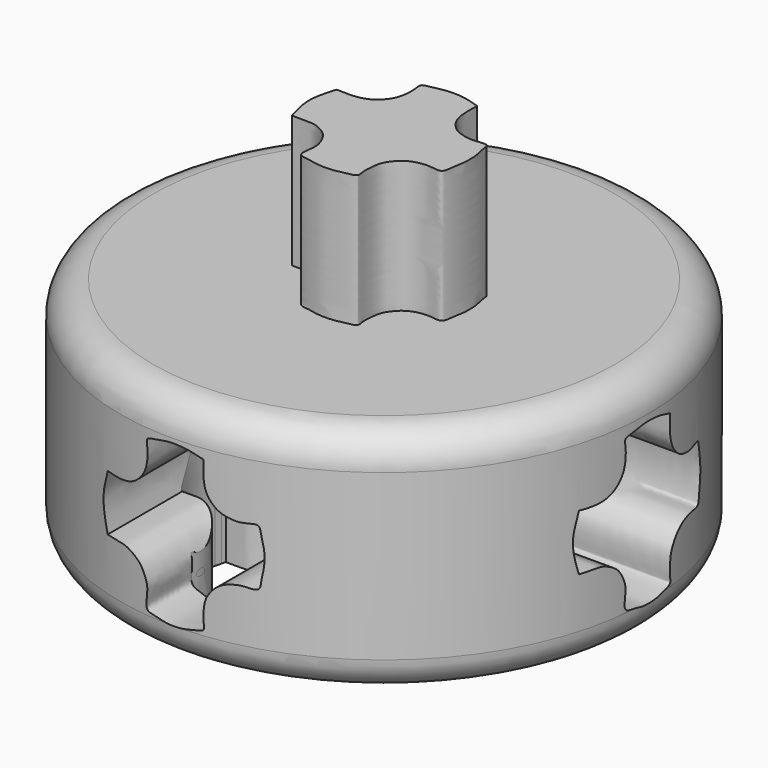
from build123d import *

# Parameters (mm, degrees)
F0_R          = 8
F1_DEPTH      = 7
F3_DEPTH      = 4
F5_DEPTH      = 25
F5_DEPTH_BACK = 25
F7_DEPTH      = 25
F7_DEPTH_BACK = 25
F9_DEPTH      = 5


# Not quite as in the source:
# - a fillet or chamfer that OpenCascade refuses, or shapes differently, is made with other operations: its cross-section is extruded or revolved along the edge and cut away or added


with BuildPart() as f1:
    # F0 (on Top) → F1 (new body)
    with BuildSketch(Plane.XY):
        Circle(F0_R)
    extrude(amount=F1_DEPTH)

    # F2 (on face) → F3 (join)
    with BuildSketch(Plane.XY.offset(7)):
        with BuildLine():
            add(Edge.make_bspline(
                [(-2.1453189292, -0.812403534), (-2.2291799027, -0.5147854162), (-2.3965988205, 0.0693154166), (-2.2270661408, 0.6183251281), (-2.1453189292, 0.8875972993)],
                knots=[0, 0, 0, 0, 0.5095712537, 1, 1, 1, 1], degree=3))
            add(Edge.make_bspline(
                [(-2.1453189292, -0.812403534), (-2.0462146869, -0.812546633), (-1.8562976232, -0.8128208589), (-1.5995258635, -0.8109702484), (-1.4107650431, -0.8271952097), (-1.0525308973, -0.9991228135), (-0.881515203, -1.2019496068), (-0.7462403154, -1.4790785152), (-0.6941521408, -1.7721486922), (-0.8264550317, -2.3060372512), (-0.4252380891, -2.3094553952), (-0.1641394597, -2.39328354), (0.171847139, -2.4065584213), (0.4619958492, -2.3819187352), (0.7053356837, -2.3086277115), (1.0355815173, -2.2738283861), (0.9578656682, -2.0264843097), (0.972329852, -1.7262282264), (1.0043166569, -1.4743095735), (1.0802938039, -1.2844806936), (1.2606264856, -1.0560642251), (1.4022161443, -0.9536037149), (1.5820445887, -0.8553488053), (1.8405387734, -0.8091796541), (2.0652910938, -0.7963302445), (2.4574534093, -0.8884051228), (2.4647792182, -0.5364288415), (2.5502262108, -0.2130675085), (2.5516869242, 0.0734966508), (2.5466202723, 0.3368604343), (2.4464405951, 0.6869113476), (2.4458836528, 0.9477445076), (2.0587086229, 0.8750622393), (1.8110087922, 0.8774528734), (1.460553932, 0.9794284484), (1.2720689076, 1.1213458505), (1.039296652, 1.3914645052), (0.9576696828, 1.8177575628), (0.969636174, 2.1409695187), (0.9758471819, 2.3087272993)],
                knots=[0, 0, 0, 0, 0.0273605905, 0.0524320947, 0.0745076412, 0.1056108167, 0.1318649214, 0.158948127, 0.1874687016, 0.220995097, 0.2482860623, 0.2755720453, 0.3045111481, 0.3315301836, 0.3578655515, 0.3837385363, 0.4059679792, 0.434252013, 0.4594532962, 0.4822711791, 0.5090972104, 0.530231005, 0.5527300135, 0.5781274322, 0.6031996615, 0.6315546276, 0.6576667534, 0.6876672756, 0.714256594, 0.7402463844, 0.7710533559, 0.7932728015, 0.8216277676, 0.8482190477, 0.8777914221, 0.9023565188, 0.9315770045, 0.9644861842, 1, 1, 1, 1], degree=3))
            add(Edge.make_bspline(
                [(-2.1453189292, 0.8875972993), (-1.9521964497, 0.8780475085), (-1.5848074134, 0.8603693676), (-1.1304602567, 0.9960226139), (-0.8202192306, 1.3400161654), (-0.7149185223, 1.6828007485), (-0.70557119, 2.0923268409), (-0.7793227574, 2.3463238004), (-0.4576002352, 2.3842425435), (-0.1008664347, 2.4800264396), (0.2451665152, 2.4783343449), (0.5684540927, 2.4417658867), (0.8334725478, 2.3546593956), (0.9758471819, 2.3087272993)],
                knots=[0, 0, 0, 0, 0.1117445823, 0.2125923647, 0.3107430927, 0.4000660841, 0.4960442665, 0.5626441507, 0.6379036869, 0.7311412958, 0.8178947498, 0.9022950941, 1, 1, 1, 1], degree=3))
        make_face()
    extrude(amount=F3_DEPTH)

    # F4 (on Right) → F5 (cut, two sides)
    with BuildSketch(Plane.YZ) as f5_sk:
        with BuildLine():
            add(Edge.make_bspline(
                [(-2.2211652576, 2.5211653882), (-2.3050262311, 2.8187835061), (-2.4724451489, 3.4028843389), (-2.3029124692, 3.9518940503), (-2.2211652576, 4.2211662216)],
                knots=[0, 0, 0, 0, 0.5095712537, 1, 1, 1, 1], degree=3))
            add(Edge.make_bspline(
                [(-2.2211652576, 2.5211653882), (-2.1220610153, 2.5210222892), (-1.9321439516, 2.5207480634), (-1.6753721919, 2.5225986738), (-1.4866113715, 2.5063737125), (-1.1283772257, 2.3344461087), (-0.9573615314, 2.1316193155), (-0.8220866438, 1.854490407), (-0.7699984692, 1.56142023), (-0.9023013601, 1.0275316711), (-0.5010844175, 1.024113527), (-0.2399857881, 0.9402853822), (0.0960008106, 0.927010501), (0.3861495208, 0.951650187), (0.6294893553, 1.0249412107), (0.9597351889, 1.0597405361), (0.8820193398, 1.3070846125), (0.8964835236, 1.6073406958), (0.9284703285, 1.8592593487), (1.0044474755, 2.0490882286), (1.1847801572, 2.2775046971), (1.3263698159, 2.3799652073), (1.5061982603, 2.478220117), (1.764692445, 2.5243892682), (1.9894447654, 2.5372386778), (2.3816070809, 2.4451637994), (2.3889328898, 2.7971400808), (2.4743798824, 3.1205014137), (2.4758405958, 3.4070655731), (2.4707739439, 3.6704293566), (2.3705942667, 4.0204802698), (2.3700373244, 4.2813134299), (1.9828622945, 4.2086311615), (1.7351624638, 4.2110217957), (1.3847076036, 4.3129973707), (1.1962225792, 4.4549147728), (0.9634503236, 4.7250334274), (0.8818233544, 5.1513264851), (0.8937898456, 5.4745384409), (0.9000008535, 5.6422962216)],
                knots=[0, 0, 0, 0, 0.0273605905, 0.0524320947, 0.0745076412, 0.1056108167, 0.1318649214, 0.158948127, 0.1874687016, 0.220995097, 0.2482860623, 0.2755720453, 0.3045111481, 0.3315301836, 0.3578655515, 0.3837385363, 0.4059679792, 0.434252013, 0.4594532962, 0.4822711791, 0.5090972104, 0.530231005, 0.5527300135, 0.5781274322, 0.6031996615, 0.6315546276, 0.6576667534, 0.6876672756, 0.714256594, 0.7402463844, 0.7710533559, 0.7932728015, 0.8216277676, 0.8482190477, 0.8777914221, 0.9023565188, 0.9315770045, 0.9644861842, 1, 1, 1, 1], degree=3))
            add(Edge.make_bspline(
                [(-2.2211652576, 4.2211662216), (-2.0280427781, 4.2116164307), (-1.6606537418, 4.1939382898), (-1.2063065851, 4.3295915362), (-0.896065559, 4.6735850876), (-0.7907648507, 5.0163696708), (-0.7814175184, 5.4258957632), (-0.8551690858, 5.6798927226), (-0.5334465636, 5.7178114657), (-0.1767127631, 5.8135953618), (0.1693201868, 5.8119032671), (0.4926077643, 5.775334809), (0.7576262194, 5.6882283179), (0.9000008535, 5.6422962216)],
                knots=[0, 0, 0, 0, 0.1117445823, 0.2125923647, 0.3107430927, 0.4000660841, 0.4960442665, 0.5626441507, 0.6379036869, 0.7311412958, 0.8178947498, 0.9022950941, 1, 1, 1, 1], degree=3))
        make_face()
    extrude(amount=-F5_DEPTH, mode=Mode.SUBTRACT)
    extrude(f5_sk.sketch, amount=F5_DEPTH_BACK, mode=Mode.SUBTRACT)

    # F6 (on Front) → F7 (cut, two sides)
    with BuildSketch(Plane.XZ) as f7_sk:
        with BuildLine():
            add(Edge.make_bspline(
                [(-2.2311653919, 2.5852779835), (-2.3150263655, 2.8828961014), (-2.4824452833, 3.4669969342), (-2.3129126036, 4.0160066456), (-2.2311653919, 4.2852788168)],
                knots=[0, 0, 0, 0, 0.5095712537, 1, 1, 1, 1], degree=3))
            add(Edge.make_bspline(
                [(-2.2311653919, 2.5852779835), (-2.1320611497, 2.5851348845), (-1.942144086, 2.5848606586), (-1.6853723262, 2.5867112691), (-1.4966115058, 2.5704863078), (-1.13837736, 2.398558704), (-0.9673616658, 2.1957319107), (-0.8320867781, 1.9186030023), (-0.7799986035, 1.6255328253), (-0.9123014945, 1.0916442664), (-0.5110845519, 1.0882261223), (-0.2499859225, 1.0043979775), (0.0860006762, 0.9911230963), (0.3761493864, 1.0157627823), (0.619489221, 1.089053806), (0.9497350545, 1.1238531314), (0.8720192055, 1.3711972078), (0.8864833893, 1.6714532911), (0.9184701942, 1.923371944), (0.9944473412, 2.1132008239), (1.1747800229, 2.3416172924), (1.3163696815, 2.4440778026), (1.496198126, 2.5423327122), (1.7546923106, 2.5885018635), (1.979444631, 2.6013512731), (2.3716069465, 2.5092763947), (2.3789327554, 2.8612526761), (2.464379748, 3.184614009), (2.4658404614, 3.4711781683), (2.4607738096, 3.7345419519), (2.3605941323, 4.0845928651), (2.3600371901, 4.3454260251), (1.9728621602, 4.2727437568), (1.7251623295, 4.275134391), (1.3747074692, 4.377109966), (1.1862224448, 4.5190273681), (0.9534501893, 4.7891460227), (0.8718232201, 5.2154390804), (0.8837897113, 5.5386510362), (0.8900007192, 5.7064088168)],
                knots=[0, 0, 0, 0, 0.0273605905, 0.0524320947, 0.0745076412, 0.1056108167, 0.1318649214, 0.158948127, 0.1874687016, 0.220995097, 0.2482860623, 0.2755720453, 0.3045111481, 0.3315301836, 0.3578655515, 0.3837385363, 0.4059679792, 0.434252013, 0.4594532962, 0.4822711791, 0.5090972104, 0.530231005, 0.5527300135, 0.5781274322, 0.6031996615, 0.6315546276, 0.6576667534, 0.6876672756, 0.714256594, 0.7402463844, 0.7710533559, 0.7932728015, 0.8216277676, 0.8482190477, 0.8777914221, 0.9023565188, 0.9315770045, 0.9644861842, 1, 1, 1, 1], degree=3))
            add(Edge.make_bspline(
                [(-2.2311653919, 4.2852788168), (-2.0380429125, 4.275729026), (-1.6706538762, 4.2580508851), (-1.2163067194, 4.3937041315), (-0.9060656934, 4.7376976829), (-0.8007649851, 5.080482266), (-0.7914176528, 5.4900083584), (-0.8651692201, 5.7440053179), (-0.5434466979, 5.781924061), (-0.1867128974, 5.8777079571), (0.1593200525, 5.8760158624), (0.4826076299, 5.8394474043), (0.7476260851, 5.7523409132), (0.8900007192, 5.7064088168)],
                knots=[0, 0, 0, 0, 0.1117445823, 0.2125923647, 0.3107430927, 0.4000660841, 0.4960442665, 0.5626441507, 0.6379036869, 0.7311412958, 0.8178947498, 0.9022950941, 1, 1, 1, 1], degree=3))
        make_face()
    extrude(amount=-F7_DEPTH, mode=Mode.SUBTRACT)
    extrude(f7_sk.sketch, amount=F7_DEPTH_BACK, mode=Mode.SUBTRACT)

    # F8 (on face) → F9 (cut)
    with BuildSketch(Plane(origin=(0, 0, 0), x_dir=(1, 0, 0), z_dir=(0, 0, -1))):
        with BuildLine():
            add(Edge.make_bspline(
                [(-2.2586211533, 3.1688635354), (-2.2701252671, 3.209691021), (-2.2816567817, 3.2505189386), (-2.2929844467, 3.2913235385)],
                knots=[0, 0, 0, 0, 0.0701518979, 0.0701518979, 0.0701518979, 0.0701518979], degree=3))
            add(Edge.make_bspline(
                [(-2.2586211533, 3.1688635354), (-2.2562431907, 3.1688601018), (-2.2538652281, 3.1688566682), (-2.2514873005, 3.1688532406)],
                knots=[0, 0, 0, 0, 0.0006588393, 0.0006588393, 0.0006588393, 0.0006588393], degree=3))
            ThreePointArc((-2.2514873005, 3.1688532406), (-2.2730608458, 3.2298088606), (-2.2929844467, 3.2913235385))
        make_face()
        with BuildLine():
            add(Edge.make_bspline(
                [(-2.2929844467, 3.2913235385), (-2.3099970518, 3.3526064717), (-2.3265498551, 3.4138368097), (-2.3418594746, 3.4749340982)],
                knots=[0.0701518979, 0.0701518979, 0.0701518979, 0.0701518979, 0.1755104625, 0.1755104625, 0.1755104625, 0.1755104625], degree=3))
            ThreePointArc((-2.2929844467, 3.2913235385), (-2.2730608458, 3.2298088606), (-2.2514873005, 3.1688532406))
            add(Edge.make_bspline(
                [(-2.2514873005, 3.1688532406), (-2.1551135176, 3.1687143242), (-1.9683612368, 3.1684639951), (-1.7147615805, 3.1702917435), (-1.5266694526, 3.1541242598), (-1.169704365, 2.9828057161), (-0.9992945004, 2.7806974445), (-0.8644988292, 2.5045502759), (-0.812595179, 2.2125183113), (-0.9041566506, 1.8430356659), (-0.8424904081, 1.7527327902)],
                knots=[0.0006588393, 0.0006588393, 0.0006588393, 0.0006588393, 0.0273605905, 0.0524320947, 0.0745076412, 0.1056108167, 0.1318649214, 0.158948127, 0.1874687016, 0.220995097, 0.220995097, 0.220995097, 0.220995097], degree=3))
            ThreePointArc((-0.8424904081, 1.7527327902), (-0.6840526351, 1.699549611), (-0.5222978031, 1.6575216106))
            add(Edge.make_bspline(
                [(-0.5222978031, 1.6575216106), (-0.4918814529, 1.6522432351), (-0.4628724934, 1.6460520009), (-0.4343789789, 1.6396367011)],
                knots=[0.2520084037, 0.2520084037, 0.2520084037, 0.2520084037, 0.2603328893, 0.2603328893, 0.2603328893, 0.2603328893], degree=3))
            ThreePointArc((-0.4343789789, 1.6396367011), (-0.2180918186, 1.6099297168), (0, 1.6))
            ThreePointArc((0, 1.6), (0.434569746, 1.6396718161), (0.8547726828, 1.7573757201))
            add(Edge.make_bspline(
                [(0.8547726828, 1.7573757201), (0.8832221623, 1.8011123631), (0.8337179729, 1.9621493035), (0.8479832374, 2.258276102), (0.8798567277, 2.5093023235), (0.9555647228, 2.6984587273), (1.135258569, 2.9260660217), (1.2763466409, 3.0281635615), (1.4555380362, 3.1260703994), (1.7131164952, 3.1720759946), (1.9298250014, 3.1844655279), (2.1747453657, 3.1289762239), (2.2475946375, 3.1583834926)],
                knots=[0.3845143326, 0.3845143326, 0.3845143326, 0.3845143326, 0.4059679792, 0.434252013, 0.4594532962, 0.4822711791, 0.5090972104, 0.530231005, 0.5527300135, 0.5781274322, 0.6031996615, 0.6290037222, 0.6290037222, 0.6290037222, 0.6290037222], degree=3))
            ThreePointArc((2.2475946375, 3.1583834926), (2.3615913205, 3.5723477639), (2.4, 4))
            ThreePointArc((2.4, 4), (2.3582082582, 4.4459302759), (2.2342884908, 4.8763303827))
            add(Edge.make_bspline(
                [(2.2342884908, 4.8763303827), (2.1630905773, 4.894204301), (1.918004699, 4.8504721227), (1.6836911252, 4.8527335616), (1.3344777647, 4.9543478842), (1.1466604558, 5.0957625385), (0.9147128049, 5.3649242874), (0.8354150914, 5.7790529149), (0.844533801, 6.088749941), (0.8502137988, 6.2443565885)],
                knots=[0.7975561416, 0.7975561416, 0.7975561416, 0.7975561416, 0.8216277676, 0.8482190477, 0.8777914221, 0.9023565188, 0.9315770045, 0.9644861842, 0.997550937, 0.997550937, 0.997550937, 0.997550937], degree=3))
            ThreePointArc((0.8502137988, 6.2443565885), (-0.0038910602, 6.3999968458), (-0.8574867585, 6.2415879325))
            add(Edge.make_bspline(
                [(-2.2398879858, 4.86191752), (-2.0537108529, 4.8527572001), (-1.69481224, 4.8372879156), (-1.2473576566, 4.9708832643), (-0.9382156713, 5.3136582053), (-0.8332879949, 5.6552284609), (-0.8245936584, 6.0361454442), (-0.8644471392, 6.1996715363), (-0.8574867585, 6.2415879325)],
                knots=[0.0036260858, 0.0036260858, 0.0036260858, 0.0036260858, 0.1117445823, 0.2125923647, 0.3107430927, 0.4000660841, 0.4960442665, 0.5458795587, 0.5458795587, 0.5458795587, 0.5458795587], degree=3))
            ThreePointArc((-2.2398879858, 4.86191752), (-2.3935398891, 4.1759738597), (-2.3418594746, 3.4749340982))
        make_face()
        with BuildLine():
            add(Edge.make_bspline(
                [(-2.3418594746, 3.4749340982), (-2.3904017419, 3.668655497), (-2.4793615243, 4.143474563), (-2.3400787723, 4.5945237862), (-2.2586211533, 4.8628420505)],
                knots=[0.1755104625, 0.1755104625, 0.1755104625, 0.1755104625, 0.5095712537, 1, 1, 1, 1], degree=3))
            ThreePointArc((-2.3418594746, 3.4749340982), (-2.3935398891, 4.1759738597), (-2.2398879858, 4.86191752))
            add(Edge.make_bspline(
                [(-2.2586211533, 4.8628420505), (-2.252376574, 4.8625332598), (-2.2461320076, 4.8622247394), (-2.2398879858, 4.86191752)],
                knots=[0, 0, 0, 0, 0.0036260858, 0.0036260858, 0.0036260858, 0.0036260858], degree=3))
        make_face()
        with BuildLine():
            ThreePointArc((0, -1.6), (-0.4359982581, -1.6399352723), (-0.8574867585, -1.7584120675))
            add(Edge.make_bspline(
                [(-2.2398879858, -3.13808248), (-2.0537108529, -3.1472427999), (-1.69481224, -3.1627120844), (-1.2473576566, -3.0291167357), (-0.9382156713, -2.6863417947), (-0.8332879949, -2.3447715391), (-0.8245936584, -1.9638545558), (-0.8644471392, -1.8003284637), (-0.8574867585, -1.7584120675)],
                knots=[0.0036260858, 0.0036260858, 0.0036260858, 0.0036260858, 0.1117445823, 0.2125923647, 0.3107430927, 0.4000660841, 0.4960442665, 0.5458795587, 0.5458795587, 0.5458795587, 0.5458795587], degree=3))
            ThreePointArc((-2.2398879858, -3.13808248), (-2.3935398891, -3.8240261403), (-2.3418594746, -4.5250659018))
            add(Edge.make_bspline(
                [(-2.2929844467, -4.7086764615), (-2.3099970518, -4.6473935283), (-2.3265498551, -4.5861631903), (-2.3418594746, -4.5250659018)],
                knots=[0.0701518979, 0.0701518979, 0.0701518979, 0.0701518979, 0.1755104625, 0.1755104625, 0.1755104625, 0.1755104625], degree=3))
            ThreePointArc((-2.2929844467, -4.7086764615), (-2.2730608458, -4.7701911395), (-2.2514873004, -4.8311467596))
            add(Edge.make_bspline(
                [(-2.2514873004, -4.8311467596), (-2.154198981, -4.8312870011), (-1.9688017614, -4.8315355561), (-1.7146679445, -4.8297083917), (-1.5267043969, -4.8458756898), (-1.1696955195, -5.0171942966), (-0.9992967723, -5.2193025522), (-0.8644981791, -5.495449725), (-0.8125953933, -5.7874816884), (-0.9041566822, -6.1569643341), (-0.8424904081, -6.2472672098)],
                knots=[0.0006591099, 0.0006591099, 0.0006591099, 0.0006591099, 0.0276362791, 0.0529604067, 0.0752583889, 0.1066749637, 0.1331936079, 0.1605497071, 0.1893576584, 0.2232218696, 0.2232218696, 0.2232218696, 0.2232218696], degree=3))
            ThreePointArc((-0.8424904081, -6.2472672098), (-0.6840526309, -6.3004503903), (-0.5222977947, -6.3424783913))
            add(Edge.make_bspline(
                [(-0.5222977947, -6.3424783913), (-0.4918814561, -6.3477567653), (-0.4628725064, -6.3539479973), (-0.4343790009, -6.3603632948)],
                knots=[0.2545476711, 0.2545476711, 0.2545476711, 0.2545476711, 0.2629560324, 0.2629560324, 0.2629560324, 0.2629560324], degree=3))
            ThreePointArc((-0.4343790009, -6.3603632948), (0.2182849751, -6.39005265), (0.8547726807, -6.2426242807))
            add(Edge.make_bspline(
                [(0.8547726807, -6.2426242807), (0.8832221792, -6.1988875939), (0.833718054, -6.0378504384), (0.8479828333, -5.7417251971), (0.8798579926, -5.4906936097), (0.9555601718, -5.3015559049), (1.1352771289, -5.0738743051), (1.2762923281, -4.9720110634), (1.4557690746, -4.873186772), (1.7121367526, -4.8310740481), (1.9332755681, -4.803873392), (2.1660968314, -4.896737202), (2.2448890949, -4.848806781)],
                knots=[0.3883887435, 0.3883887435, 0.3883887435, 0.3883887435, 0.4100585604, 0.4386275875, 0.4640828018, 0.4871306004, 0.5142269339, 0.5355736752, 0.5582993863, 0.5839527124, 0.6092775725, 0.6352778184, 0.6352778184, 0.6352778184, 0.6352778184], degree=3))
            ThreePointArc((2.2448890949, -4.848806781), (2.2910988522, -4.7147489414), (2.3293109061, -4.5781960764))
            add(Edge.make_bspline(
                [(2.3293109061, -4.5781960764), (2.318320841, -4.5478681347), (2.3650244047, -4.3109120088), (2.397358483, -4.1125713275)],
                knots=[0.6723774853, 0.6723774853, 0.6723774853, 0.6723774853, 0.7023456049, 0.7023456049, 0.7023456049, 0.7023456049], degree=3))
            ThreePointArc((2.397358483, -4.1125713275), (2.3993395299, -4.0563011576), (2.4, -4))
            ThreePointArc((2.4, -4), (2.3582499283, -3.5542901441), (2.2344522703, -3.1240873036))
            add(Edge.make_bspline(
                [(2.2344522703, -3.1240873036), (2.1631307294, -3.1065494653), (1.9182298235, -3.1491156388), (1.6836489231, -3.1473942735), (1.3344869446, -3.0456331454), (1.1466588745, -2.9042117851), (0.9147076065, -2.6352385745), (0.8354228453, -2.2201500831), (0.8444835984, -1.9125641254), (0.8502136413, -1.7556433518)],
                knots=[0.7954847882, 0.7954847882, 0.7954847882, 0.7954847882, 0.8198304679, 0.8466896849, 0.8765600341, 0.9013726516, 0.9308875663, 0.9641283428, 0.9975481171, 0.9975481171, 0.9975481171, 0.9975481171], degree=3))
            ThreePointArc((0.8502136413, -1.7556433518), (0.4321712881, -1.6392314858), (0, -1.6))
        make_face()
    extrude(amount=-F9_DEPTH, mode=Mode.SUBTRACT)

    # F10: fillet of radius 1 on 2 edges, made by hand

    # F10_s1 → F10_t2 (revolve, cut)
    with BuildSketch(Plane.XZ):
        with BuildLine():
            ThreePointArc((8, 1), (7.7071067812, 0.2928932188), (7, 0))
            Line((7, 0), (8, 0))
            Line((8, 0), (8, 1))
        make_face()
    revolve(axis=Axis((0, 0, 0), (0, 0, 1)), mode=Mode.SUBTRACT)

    # F10_s3 → F10_t4 (revolve, cut)
    with BuildSketch(Plane.XZ):
        with BuildLine():
            ThreePointArc((8, 6), (7.7071067812, 6.7071067812), (7, 7))
            Line((7, 7), (8, 7))
            Line((8, 7), (8, 6))
        make_face()
    revolve(axis=Axis((0, 0, 7), (0, 0, 1)), mode=Mode.SUBTRACT)


solid = f1.part
